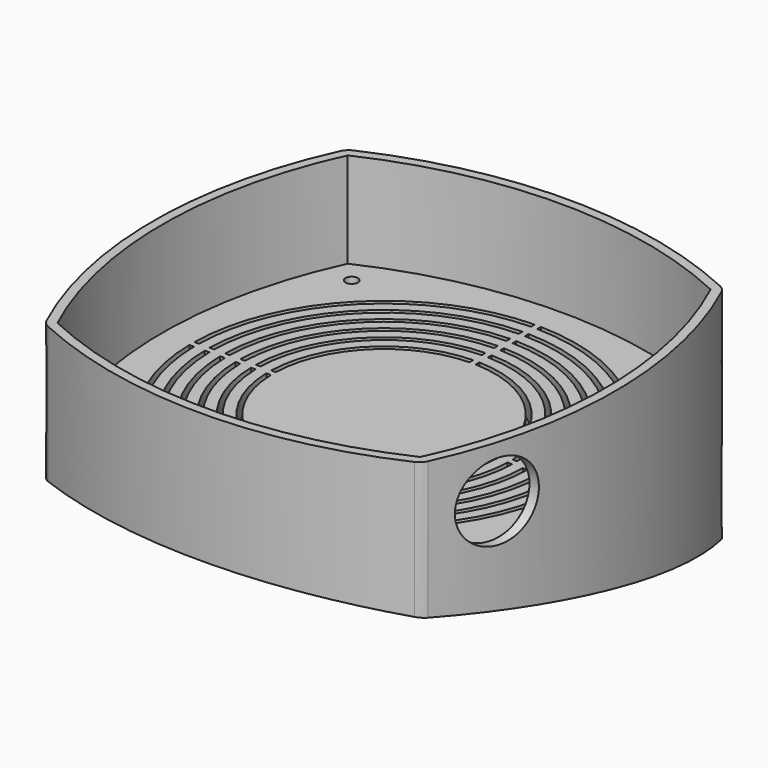
from build123d import *

# Parameters (mm, degrees)
F1_DEPTH        = 80
F2_R            = 1379.3418086479
F3_DEPTH        = 390
F0_R            = 47.8625
F7_DEPTH        = 40
F8_R            = 47.8625
F10_R           = 42.8625
F11_DEPTH       = 3
F14_DEPTH       = 31
F16_DEPTH       = 25
F17_R           = 5
F20_D           = 4
F20_START       = 24.8328661
F20_CBORE_D     = 8
F20_CBORE_DEPTH = 5
F21_R           = 2
F22_DEPTH       = 3
F23_R           = 12.5
F24_DEPTH       = 249
F25_R           = 125
F26_DEPTH       = 94


# Not quite as in the source:
# - a feature names something its author has since deleted; it is built from what else it names


with BuildPart() as f1:
    # F0 (on Top) → F1 (new body, symmetric)
    with BuildSketch(Plane.XY):
        with BuildLine():
            ThreePointArc((61.2553872941, -61.2553872941), (75.039376183, 0), (61.2553872941, 61.2553872941))
            ThreePointArc((61.2553872941, 61.2553872941), (0, 75.039376183), (-61.2553872941, 61.2553872941))
            ThreePointArc((-61.2553872941, 61.2553872941), (-75.039376183, 0), (-61.2553872941, -61.2553872941))
            ThreePointArc((-61.2553872941, -61.2553872941), (0, -75.039376183), (61.2553872941, -61.2553872941))
        make_face()
        with BuildLine():
            ThreePointArc((-59, 59), (0, 72.039376183), (59, 59))
            ThreePointArc((59, 59), (72.039376183, 0), (59, -59))
            ThreePointArc((59, -59), (0, -72.039376183), (-59, -59))
            ThreePointArc((-59, -59), (-72.039376183, 0), (-59, 59))
        make_face(mode=Mode.SUBTRACT)
    extrude(amount=F1_DEPTH, both=True)

    # F2 (on Right) → F3 (cut, symmetric)
    with BuildSketch(Plane.YZ):
        with Locations((-294.0411567688, 1407.0612192154)):
            Circle(F2_R)
        with Locations((-294.0411567688, -1407.0612192154)):
            Circle(F2_R)
    extrude(amount=F3_DEPTH, both=True, mode=Mode.SUBTRACT)

    # F6 (on Top) + F0 (on Top) → F7 (join, symmetric)
    with BuildSketch(Plane.XY):
        with BuildLine():
            ThreePointArc((61.2553872941, -61.2553872941), (75.039376183, 0), (61.2553872941, 61.2553872941))
            ThreePointArc((61.2553872941, 61.2553872941), (0, 75.039376183), (-61.2553872941, 61.2553872941))
            ThreePointArc((-61.2553872941, 61.2553872941), (-75.039376183, 0), (-61.2553872941, -61.2553872941))
            ThreePointArc((-61.2553872941, -61.2553872941), (0, -75.039376183), (61.2553872941, -61.2553872941))
        make_face()
        with BuildLine():
            ThreePointArc((-59, 59), (0, 72.039376183), (59, 59))
            ThreePointArc((59, 59), (72.039376183, 0), (59, -59))
            ThreePointArc((59, -59), (0, -72.039376183), (-59, -59))
            ThreePointArc((-59, -59), (-72.039376183, 0), (-59, 59))
        make_face(mode=Mode.SUBTRACT)
        with BuildLine():
            ThreePointArc((59, -59), (72.039376183, 0), (59, 59))
            ThreePointArc((59, 59), (0, 72.039376183), (-59, 59))
            ThreePointArc((-59, 59), (-72.039376183, 0), (-59, -59))
            ThreePointArc((-59, -59), (0, -72.039376183), (59, -59))
        make_face()
    with BuildSketch(Plane.XY):
        with BuildLine():
            ThreePointArc((59, -59), (72.039376183, 0), (59, 59))
            ThreePointArc((59, 59), (0, 72.039376183), (-59, 59))
            ThreePointArc((-59, 59), (-72.039376183, 0), (-59, -59))
            ThreePointArc((-59, -59), (0, -72.039376183), (59, -59))
        make_face()
        Circle(F0_R, mode=Mode.SUBTRACT)
    extrude(amount=F7_DEPTH, both=True)

    # F5 (on offset) → F9 section 0
    with BuildSketch(Plane.XY.offset(40)):
        with BuildLine():
            ThreePointArc((59, -59), (72.039376183, 0), (59, 59))
            ThreePointArc((59, 59), (0, 72.039376183), (-59, 59))
            ThreePointArc((-59, 59), (-72.039376183, 0), (-59, -59))
            ThreePointArc((-59, -59), (0, -72.039376183), (59, -59))
        make_face()
    # F8 (on Top) → F9 section 1
    with BuildSketch(Plane.XY):
        Circle(F8_R)
    loft(mode=Mode.SUBTRACT)

    # F10 (on face) → F11 (cut)
    with BuildSketch(Plane.XY):
        Circle(F10_R)
    extrude(amount=-F11_DEPTH, mode=Mode.SUBTRACT)

    # F13 (on offset) → F14 (cut)
    with BuildSketch(Plane.XY.offset(-3)):
        with BuildLine():
            ThreePointArc((59, -59), (72.039376183, 0), (59, 59))
            ThreePointArc((59, 59), (0, 72.039376183), (-59, 59))
            ThreePointArc((-59, 59), (-72.039376183, 0), (-59, -59))
            ThreePointArc((-59, -59), (0, -72.039376183), (59, -59))
        make_face()
    extrude(amount=-F14_DEPTH, mode=Mode.SUBTRACT)

    # F15 (on face) → F16 (cut)
    with BuildSketch(Plane(origin=(0, 0, -40), x_dir=(1, 0, 0), z_dir=(0, 0, -1))):
        with BuildLine():
            Line((-1, 60.9918027279), (-1, 62.4919994879))
            ThreePointArc((-1, 62.4919994879), (-44.1941738242, 44.1941738242), (-62.4919994879, 1))
            Line((-62.4919994879, 1), (-60.9918027279, 1))
            ThreePointArc((-60.9918027279, 1), (-43.1335136524, 43.1335136524), (-1, 60.9918027279))
        make_face()
        with BuildLine():
            Line((-1, 55.9910707167), (-1, 57.4913036902))
            ThreePointArc((-1, 57.4913036902), (-40.6586399182, 40.6586399182), (-57.4913036902, 1))
            Line((-57.4913036902, 1), (-55.9910707167, 1))
            ThreePointArc((-55.9910707167, 1), (-39.5979797464, 39.5979797464), (-1, 55.9910707167))
        make_face()
        with BuildLine():
            Line((-1, 50.9901951359), (-1, 52.4904753265))
            ThreePointArc((-1, 52.4904753265), (-37.1231060123, 37.1231060123), (-52.4904753265, 1))
            Line((-52.4904753265, 1), (-50.9901951359, 1))
            ThreePointArc((-50.9901951359, 1), (-36.0624458405, 36.0624458405), (-1, 50.9901951359))
        make_face()
        with BuildLine():
            Line((-1, 45.9891291503), (-1, 47.4894725176))
            ThreePointArc((-1, 47.4894725176), (-33.5875721064, 33.5875721064), (-47.4894725176, 1))
            Line((-47.4894725176, 1), (-45.9891291503, 1))
            ThreePointArc((-45.9891291503, 1), (-32.5269119346, 32.5269119346), (-1, 45.9891291503))
        make_face()
        with BuildLine():
            Line((-1, 40.9878030638), (-1, 42.4882336653))
            ThreePointArc((-1, 42.4882336653), (-30.0520382004, 30.0520382004), (-42.4882336653, 1))
            Line((-42.4882336653, 1), (-40.9878030638, 1))
            ThreePointArc((-40.9878030638, 1), (-28.9913780286, 28.9913780286), (-1, 40.9878030638))
        make_face()
        with BuildLine():
            Line((-1, 35.9861084309), (-1, 37.4866642955))
            ThreePointArc((-1, 37.4866642955), (-26.5165042945, 26.5165042945), (-37.4866642955, 1))
            Line((-37.4866642955, 1), (-35.9861084309, 1))
            ThreePointArc((-35.9861084309, 1), (-25.4558441227, 25.4558441227), (-1, 35.9861084309))
        make_face()
        with BuildLine():
            Line((35.9861084309, 1), (37.4866642955, 1))
            ThreePointArc((37.4866642955, 1), (26.5165042945, 26.5165042945), (1, 37.4866642955))
            Line((1, 37.4866642955), (1, 35.9861084309))
            ThreePointArc((1, 35.9861084309), (25.4558441227, 25.4558441227), (35.9861084309, 1))
        make_face()
        with BuildLine():
            Line((40.9878030638, 1), (42.4882336653, 1))
            ThreePointArc((42.4882336653, 1), (30.0520382004, 30.0520382004), (1, 42.4882336653))
            Line((1, 42.4882336653), (1, 40.9878030638))
            ThreePointArc((1, 40.9878030638), (28.9913780286, 28.9913780286), (40.9878030638, 1))
        make_face()
        with BuildLine():
            Line((45.9891291503, 1), (47.4894725176, 1))
            ThreePointArc((47.4894725176, 1), (33.5875721064, 33.5875721064), (1, 47.4894725176))
            Line((1, 47.4894725176), (1, 45.9891291503))
            ThreePointArc((1, 45.9891291503), (32.5269119346, 32.5269119346), (45.9891291503, 1))
        make_face()
        with BuildLine():
            Line((50.9901951359, 1), (52.4904753265, 1))
            ThreePointArc((52.4904753265, 1), (37.1231060123, 37.1231060123), (1, 52.4904753265))
            Line((1, 52.4904753265), (1, 50.9901951359))
            ThreePointArc((1, 50.9901951359), (36.0624458405, 36.0624458405), (50.9901951359, 1))
        make_face()
        with BuildLine():
            Line((55.9910707167, 1), (57.4913036902, 1))
            ThreePointArc((57.4913036902, 1), (40.6586399182, 40.6586399182), (1, 57.4913036902))
            Line((1, 57.4913036902), (1, 55.9910707167))
            ThreePointArc((1, 55.9910707167), (39.5979797464, 39.5979797464), (55.9910707167, 1))
        make_face()
        with BuildLine():
            Line((60.9918027279, 1), (62.4919994879, 1))
            ThreePointArc((62.4919994879, 1), (44.1941738242, 44.1941738242), (1, 62.4919994879))
            Line((1, 62.4919994879), (1, 60.9918027279))
            ThreePointArc((1, 60.9918027279), (43.1335136524, 43.1335136524), (60.9918027279, 1))
        make_face()
        with BuildLine():
            ThreePointArc((1, -37.4866642955), (26.5165042945, -26.5165042945), (37.4866642955, -1))
            Line((37.4866642955, -1), (35.9861084309, -1))
            ThreePointArc((35.9861084309, -1), (25.4558441227, -25.4558441227), (1, -35.9861084309))
            Line((1, -35.9861084309), (1, -37.4866642955))
        make_face()
        with BuildLine():
            ThreePointArc((-37.4866642955, -1), (-26.5165042945, -26.5165042945), (-1, -37.4866642955))
            Line((-1, -37.4866642955), (-1, -35.9861084309))
            ThreePointArc((-1, -35.9861084309), (-25.4558441227, -25.4558441227), (-35.9861084309, -1))
            Line((-35.9861084309, -1), (-37.4866642955, -1))
        make_face()
        with BuildLine():
            ThreePointArc((-42.4882336653, -1), (-30.0520382004, -30.0520382004), (-1, -42.4882336653))
            Line((-1, -42.4882336653), (-1, -40.9878030638))
            ThreePointArc((-1, -40.9878030638), (-28.9913780286, -28.9913780286), (-40.9878030638, -1))
            Line((-40.9878030638, -1), (-42.4882336653, -1))
        make_face()
        with BuildLine():
            ThreePointArc((1, -42.4882336653), (30.0520382004, -30.0520382004), (42.4882336653, -1))
            Line((42.4882336653, -1), (40.9878030638, -1))
            ThreePointArc((40.9878030638, -1), (28.9913780286, -28.9913780286), (1, -40.9878030638))
            Line((1, -40.9878030638), (1, -42.4882336653))
        make_face()
        with BuildLine():
            ThreePointArc((1, -47.4894725176), (33.5875721064, -33.5875721064), (47.4894725176, -1))
            Line((47.4894725176, -1), (45.9891291503, -1))
            ThreePointArc((45.9891291503, -1), (32.5269119346, -32.5269119346), (1, -45.9891291503))
            Line((1, -45.9891291503), (1, -47.4894725176))
        make_face()
        with BuildLine():
            ThreePointArc((-47.4894725176, -1), (-33.5875721064, -33.5875721064), (-1, -47.4894725176))
            Line((-1, -47.4894725176), (-1, -45.9891291503))
            ThreePointArc((-1, -45.9891291503), (-32.5269119346, -32.5269119346), (-45.9891291503, -1))
            Line((-45.9891291503, -1), (-47.4894725176, -1))
        make_face()
        with BuildLine():
            ThreePointArc((-52.4904753265, -1), (-37.1231060123, -37.1231060123), (-1, -52.4904753265))
            Line((-1, -52.4904753265), (-1, -50.9901951359))
            ThreePointArc((-1, -50.9901951359), (-36.0624458405, -36.0624458405), (-50.9901951359, -1))
            Line((-50.9901951359, -1), (-52.4904753265, -1))
        make_face()
        with BuildLine():
            ThreePointArc((1, -52.4904753265), (37.1231060123, -37.1231060123), (52.4904753265, -1))
            Line((52.4904753265, -1), (50.9901951359, -1))
            ThreePointArc((50.9901951359, -1), (36.0624458405, -36.0624458405), (1, -50.9901951359))
            Line((1, -50.9901951359), (1, -52.4904753265))
        make_face()
        with BuildLine():
            ThreePointArc((1, -57.4913036902), (40.6586399182, -40.6586399182), (57.4913036902, -1))
            Line((57.4913036902, -1), (55.9910707167, -1))
            ThreePointArc((55.9910707167, -1), (39.5979797464, -39.5979797464), (1, -55.9910707167))
            Line((1, -55.9910707167), (1, -57.4913036902))
        make_face()
        with BuildLine():
            ThreePointArc((-57.4913036902, -1), (-40.6586399182, -40.6586399182), (-1, -57.4913036902))
            Line((-1, -57.4913036902), (-1, -55.9910707167))
            ThreePointArc((-1, -55.9910707167), (-39.5979797464, -39.5979797464), (-55.9910707167, -1))
            Line((-55.9910707167, -1), (-57.4913036902, -1))
        make_face()
        with BuildLine():
            ThreePointArc((-62.4919994879, -1), (-44.1941738242, -44.1941738242), (-1, -62.4919994879))
            Line((-1, -62.4919994879), (-1, -60.9918027279))
            ThreePointArc((-1, -60.9918027279), (-43.1335136524, -43.1335136524), (-60.9918027279, -1))
            Line((-60.9918027279, -1), (-62.4919994879, -1))
        make_face()
        with BuildLine():
            ThreePointArc((1, -62.4919994879), (44.1941738242, -44.1941738242), (62.4919994879, -1))
            Line((62.4919994879, -1), (60.9918027279, -1))
            ThreePointArc((60.9918027279, -1), (43.1335136524, -43.1335136524), (1, -60.9918027279))
            Line((1, -60.9918027279), (1, -62.4919994879))
        make_face()
    extrude(amount=-F16_DEPTH, mode=Mode.SUBTRACT)

    # F17
    f17_edges = [f1.edges().sort_by_distance(p)[0] for p in [
        (-61.255387, 61.255387, 0),
        (-61.255387, -61.255387, 0),
        (61.255387, 61.255387, 0),
        (61.255387, -61.255387, 0),
        (-59, 59, 56.832446),
        (59, 59, 56.832446),
        (-59, -59, 43.946273),
        (59, -59, 43.946273),
        (59, -59, -43.946273),
        (-59, -59, -43.946273),
        (-59, 59, -56.832446),
        (59, 59, -56.832446),
    ]]
    fillet(f17_edges, radius=F17_R)

    # F20 (through all)
    # its depths count from where the whole tool has entered the part; down to there all is cleared
    with Locations(Plane.XY.offset(50).offset(-F20_START)):
        with Locations((-52.5, 52.5), (52.5, 52.5), (52.5, -52.5), (-52.5, -52.5)):
            CounterBoreHole(F20_D / 2, F20_CBORE_D / 2, F20_CBORE_DEPTH)

    # F21 (on face) → F22 (cut)
    with BuildSketch(Plane(origin=(0, 0, -40), x_dir=(1, 0, 0), z_dir=(0, 0, -1))):
        Polygon((-50.7679491924, 55.5), (-54.2320508076, 55.5), (-55.9641016151, 52.5), (-54.2320508076, 49.5), (-50.7679491924, 49.5), (-49.0358983849, 52.5), align=None)
        with Locations((-52.5, 52.5)):
            Circle(F21_R, mode=Mode.SUBTRACT)
        Polygon((54.2320508076, 55.5), (50.7679491924, 55.5), (49.0358983849, 52.5), (50.7679491924, 49.5), (54.2320508076, 49.5), (55.9641016151, 52.5), align=None)
        with Locations((52.5, 52.5)):
            Circle(F21_R, mode=Mode.SUBTRACT)
        Polygon((54.2320508076, -49.5), (50.7679491924, -49.5), (49.0358983849, -52.5), (50.7679491924, -55.5), (54.2320508076, -55.5), (55.9641016151, -52.5), align=None)
        with Locations((52.5, -52.5)):
            Circle(F21_R, mode=Mode.SUBTRACT)
        Polygon((-50.7679491924, -49.5), (-54.2320508076, -49.5), (-55.9641016151, -52.5), (-54.2320508076, -55.5), (-50.7679491924, -55.5), (-49.0358983849, -52.5), align=None)
        with Locations((-52.5, -52.5)):
            Circle(F21_R, mode=Mode.SUBTRACT)
    extrude(amount=-F22_DEPTH, mode=Mode.SUBTRACT)

    # F23 (on Right) → F24 (cut)
    with BuildSketch(Plane.YZ):
        with Locations((-40, -20)):
            Circle(F23_R)
    extrude(amount=F24_DEPTH, mode=Mode.SUBTRACT)

    # F25 (on offset) → F26 (cut)
    with BuildSketch(Plane.XY.offset(-3)):
        Circle(F25_R)
    extrude(amount=F26_DEPTH, mode=Mode.SUBTRACT)


solid = f1.part
